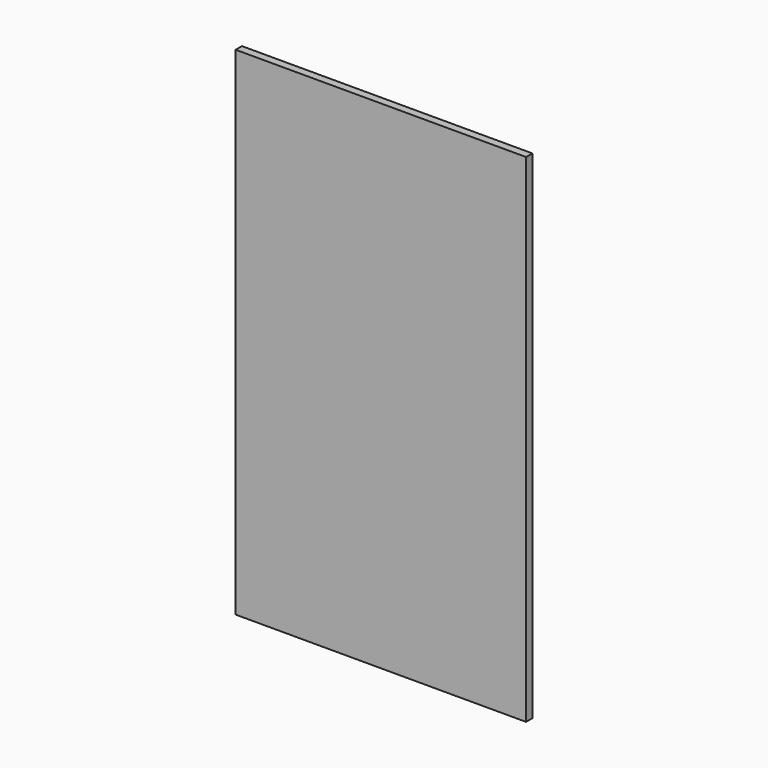
from build123d import *

# Parameters (mm, degrees)
F0_W     = 584.2
F0_H     = 1000.125
F1_DEPTH = 7.9375


# Not quite as in the source:
# - a length typed as a fraction of an inch, garbled in the dataset ("3 / 203.2 mm" for 3/8 in), is restored


with BuildPart() as f1:
    # F0 (on Front) → F1 (new body, symmetric)
    with BuildSketch(Plane.XZ):
        Rectangle(F0_W, F0_H)
    extrude(amount=F1_DEPTH, both=True)


solid = f1.part
